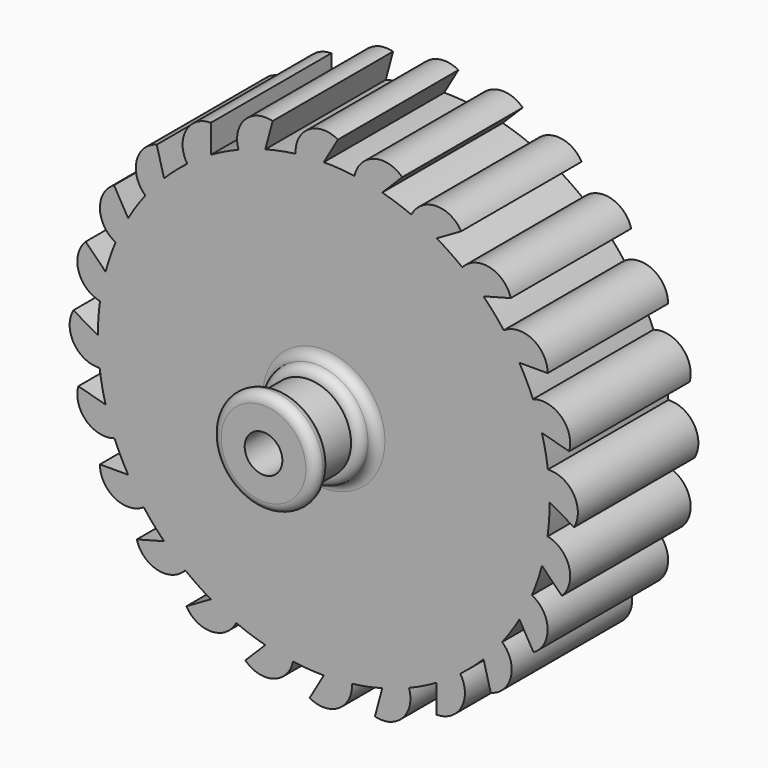
from build123d import *

# Parameters (mm, degrees)
F1_DEPTH  = 50.8
F2_R      = 17.4625
F3_DEPTH  = 6.35
F4_R      = 14.2875
F5_DEPTH  = 12.7
F6_R      = 17.4625
F7_DEPTH  = 6.35
F8_R      = 3.17499
F9_R      = 6.35
F10_DEPTH = 76.201
F11_DEPTH = 25.4


# Not quite as in the source:
# - a fillet or chamfer is up to 0.001 mm smaller than in the source, because OpenCascade refuses the exact size


with BuildPart() as f1:
    # F0 (on Front) → F1 (new body)
    with BuildSketch(Plane.XZ):
        with BuildLine():
            ThreePointArc((-56.346788131, 63.0819802218), (-63.1545591102, 56.0579284352), (-60.182611768, 46.7385626735))
            ThreePointArc((-60.182611768, 46.7385626735), (-63.234562014, 42.5185861347), (-65.9911357684, 38.1))
            Line((-65.9911357684, 38.1), (-70.7536357684, 46.348891971))
            ThreePointArc((-70.7536357684, 46.348891971), (-75.5114792005, 37.8021981611), (-70.2287691608, 29.5695786604))
            ThreePointArc((-70.2287691608, 29.5695786604), (-72.0845164259, 24.7034914868), (-73.6035479632, 19.7220112368))
            Line((-73.6035479632, 19.7220112368), (-80.338740054, 26.4572033276))
            ThreePointArc((-80.338740054, 26.4572033276), (-82.7224167718, 16.9703105533), (-75.4889519939, 10.3854767276))
            ThreePointArc((-75.4889519939, 10.3854767276), (-76.0220301687, 5.2048947186), (-76.2, 0))
            Line((-76.2, 0), (-84.448891971, 4.7625))
            ThreePointArc((-84.448891971, 4.7625), (-84.2959583455, -5.0180756738), (-75.6046875, -9.5063782813))
            ThreePointArc((-75.6046875, -9.5063782813), (-74.7787681878, -14.6484070232), (-73.6035479632, -19.7220112368))
            Line((-73.6035479632, -19.7220112368), (-82.8039914586, -17.2567598322))
            ThreePointArc((-82.8039914586, -17.2567598322), (-80.1248696635, -26.6644883366), (-70.5680884956, -28.7503893204))
            ThreePointArc((-70.5680884956, -28.7503893204), (-68.4394567327, -33.503444034), (-65.9911357684, -38.1))
            Line((-65.9911357684, -38.1), (-75.5161357684, -38.1))
            ThreePointArc((-75.5161357684, -38.1), (-70.4934035266, -46.4937601844), (-60.7223908795, -46.0351088396))
            ThreePointArc((-60.7223908795, -46.0351088396), (-57.4361094027, -50.075276701), (-53.8815367264, -53.8815367264))
            Line((-53.8815367264, -53.8815367264), (-63.0819802218, -56.346788131))
            ThreePointArc((-63.0819802218, -56.346788131), (-56.0579284352, -63.1545591102), (-46.7385626735, -60.182611768))
            ThreePointArc((-46.7385626735, -60.182611768), (-42.5185861347, -63.234562014), (-38.1, -65.9911357684))
            Line((-38.1, -65.9911357684), (-46.348891971, -70.7536357684))
            ThreePointArc((-46.348891971, -70.7536357684), (-37.8021981611, -75.5114792005), (-29.5695786604, -70.2287691608))
            ThreePointArc((-29.5695786604, -70.2287691608), (-24.7034914868, -72.0845164259), (-19.7220112368, -73.6035479632))
            Line((-19.7220112368, -73.6035479632), (-26.4572033276, -80.338740054))
            ThreePointArc((-26.4572033276, -80.338740054), (-16.9703105533, -82.7224167718), (-10.3854767276, -75.4889519939))
            ThreePointArc((-10.3854767276, -75.4889519939), (-5.2048947186, -76.0220301687), (0, -76.2))
            Line((0, -76.2), (-4.7625, -84.448891971))
            ThreePointArc((-4.7625, -84.448891971), (5.0180756738, -84.2959583455), (9.5063782813, -75.6046875))
            ThreePointArc((9.5063782813, -75.6046875), (14.6484070232, -74.7787681878), (19.7220112368, -73.6035479632))
            Line((19.7220112368, -73.6035479632), (17.2567598322, -82.8039914586))
            ThreePointArc((17.2567598322, -82.8039914586), (26.6644883366, -80.1248696635), (28.7503893204, -70.5680884956))
            ThreePointArc((28.7503893204, -70.5680884956), (33.503444034, -68.4394567327), (38.1, -65.9911357684))
            Line((38.1, -65.9911357684), (38.1, -75.5161357684))
            ThreePointArc((38.1, -75.5161357684), (46.4937601844, -70.4934035266), (46.0351088396, -60.7223908795))
            ThreePointArc((46.0351088396, -60.7223908795), (50.075276701, -57.4361094027), (53.8815367264, -53.8815367264))
            Line((53.8815367264, -53.8815367264), (56.346788131, -63.0819802218))
            ThreePointArc((56.346788131, -63.0819802218), (63.1545591102, -56.0579284352), (60.182611768, -46.7385626735))
            ThreePointArc((60.182611768, -46.7385626735), (63.234562014, -42.5185861347), (65.9911357684, -38.1))
            Line((65.9911357684, -38.1), (70.7536357684, -46.348891971))
            ThreePointArc((70.7536357684, -46.348891971), (75.5114792005, -37.8021981611), (70.2287691608, -29.5695786604))
            ThreePointArc((70.2287691608, -29.5695786604), (72.0845164259, -24.7034914868), (73.6035479632, -19.7220112368))
            Line((73.6035479632, -19.7220112368), (80.338740054, -26.4572033276))
            ThreePointArc((80.338740054, -26.4572033276), (82.7224167718, -16.9703105533), (75.4889519939, -10.3854767276))
            ThreePointArc((75.4889519939, -10.3854767276), (76.0220301687, -5.2048947186), (76.2, 0))
            Line((76.2, 0), (84.448891971, -4.7625))
            ThreePointArc((84.448891971, -4.7625), (84.2959583455, 5.0180756738), (75.6046875, 9.5063782813))
            ThreePointArc((75.6046875, 9.5063782813), (74.7787681878, 14.6484070232), (73.6035479632, 19.7220112368))
            Line((73.6035479632, 19.7220112368), (82.8039914586, 17.2567598322))
            ThreePointArc((82.8039914586, 17.2567598322), (80.1248696635, 26.6644883366), (70.5680884956, 28.7503893204))
            ThreePointArc((70.5680884956, 28.7503893204), (68.4394567327, 33.503444034), (65.9911357684, 38.1))
            Line((65.9911357684, 38.1), (75.5161357684, 38.1))
            ThreePointArc((75.5161357684, 38.1), (70.4934035266, 46.4937601844), (60.7223908795, 46.0351088396))
            ThreePointArc((60.7223908795, 46.0351088396), (57.4361094027, 50.075276701), (53.8815367264, 53.8815367264))
            Line((53.8815367264, 53.8815367264), (63.0819802218, 56.346788131))
            ThreePointArc((63.0819802218, 56.346788131), (56.0579284352, 63.1545591102), (46.7385626735, 60.182611768))
            ThreePointArc((46.7385626735, 60.182611768), (42.5185861347, 63.234562014), (38.1, 65.9911357684))
            Line((38.1, 65.9911357684), (46.348891971, 70.7536357684))
            ThreePointArc((46.348891971, 70.7536357684), (37.8021981611, 75.5114792005), (29.5695786604, 70.2287691608))
            ThreePointArc((29.5695786604, 70.2287691608), (24.7034914868, 72.0845164259), (19.7220112368, 73.6035479632))
            Line((19.7220112368, 73.6035479632), (26.4572033276, 80.338740054))
            ThreePointArc((26.4572033276, 80.338740054), (16.9703105533, 82.7224167718), (10.3854767276, 75.4889519939))
            ThreePointArc((10.3854767276, 75.4889519939), (5.2048947186, 76.0220301687), (0, 76.2))
            Line((0, 76.2), (4.7625, 84.448891971))
            ThreePointArc((4.7625, 84.448891971), (-5.0180756738, 84.2959583455), (-9.5063782813, 75.6046875))
            ThreePointArc((-9.5063782813, 75.6046875), (-14.6484070232, 74.7787681878), (-19.7220112368, 73.6035479632))
            Line((-19.7220112368, 73.6035479632), (-17.2567598322, 82.8039914586))
            ThreePointArc((-17.2567598322, 82.8039914586), (-26.6644883366, 80.1248696635), (-28.7503893204, 70.5680884956))
            ThreePointArc((-28.7503893204, 70.5680884956), (-33.503444034, 68.4394567327), (-38.1, 65.9911357684))
            Line((-38.1, 65.9911357684), (-38.1, 75.5161357684))
            ThreePointArc((-38.1, 75.5161357684), (-46.4937601844, 70.4934035266), (-46.0351088396, 60.7223908795))
            ThreePointArc((-46.0351088396, 60.7223908795), (-50.075276701, 57.4361094027), (-53.8815367264, 53.8815367264))
            Line((-53.8815367264, 53.8815367264), (-56.346788131, 63.0819802218))
        make_face()
    extrude(amount=F1_DEPTH)

    # F2 (on face) → F3 (join)
    with BuildSketch(Plane.XZ.offset(50.8)):
        Circle(F2_R)
    extrude(amount=F3_DEPTH)

    # F4 (on face) → F5 (join)
    with BuildSketch(Plane.XZ.offset(57.15)):
        Circle(F4_R)
    extrude(amount=F5_DEPTH)

    # F6 (on face) → F7 (join)
    with BuildSketch(Plane.XZ.offset(69.85)):
        Circle(F6_R)
    extrude(amount=F7_DEPTH)

    # F8 (radius 3.175 in the source; OpenCascade refuses exactly that, so slightly less here)
    f8_edges = [f1.edges().sort_by_distance(p)[0] for p in [
        (17.4625, -53.975, 0),
        (-17.4625, -50.8, 0),
        (-17.4625, -57.15, 0),
        (17.4625, -73.025, 0),
        (-17.4625, -69.85, 0),
        (-17.4625, -76.2, 0),
    ]]
    fillet(f8_edges, radius=F8_R)

    # F9 (on face) → F10 (cut, through all)
    with BuildSketch(Plane.XZ.offset(76.2)):
        Circle(F9_R)
    extrude(amount=-F10_DEPTH, mode=Mode.SUBTRACT)

    # F0 (on Front) → F11 (join)
    with BuildSketch(Plane.XZ):
        with BuildLine():
            ThreePointArc((-56.346788131, 63.0819802218), (-63.1545591102, 56.0579284352), (-60.182611768, 46.7385626735))
            ThreePointArc((-60.182611768, 46.7385626735), (-63.234562014, 42.5185861347), (-65.9911357684, 38.1))
            Line((-65.9911357684, 38.1), (-70.7536357684, 46.348891971))
            ThreePointArc((-70.7536357684, 46.348891971), (-75.5114792005, 37.8021981611), (-70.2287691608, 29.5695786604))
            ThreePointArc((-70.2287691608, 29.5695786604), (-72.0845164259, 24.7034914868), (-73.6035479632, 19.7220112368))
            Line((-73.6035479632, 19.7220112368), (-80.338740054, 26.4572033276))
            ThreePointArc((-80.338740054, 26.4572033276), (-82.7224167718, 16.9703105533), (-75.4889519939, 10.3854767276))
            ThreePointArc((-75.4889519939, 10.3854767276), (-76.0220301687, 5.2048947186), (-76.2, 0))
            Line((-76.2, 0), (-84.448891971, 4.7625))
            ThreePointArc((-84.448891971, 4.7625), (-84.2959583455, -5.0180756738), (-75.6046875, -9.5063782813))
            ThreePointArc((-75.6046875, -9.5063782813), (-74.7787681878, -14.6484070232), (-73.6035479632, -19.7220112368))
            Line((-73.6035479632, -19.7220112368), (-82.8039914586, -17.2567598322))
            ThreePointArc((-82.8039914586, -17.2567598322), (-80.1248696635, -26.6644883366), (-70.5680884956, -28.7503893204))
            ThreePointArc((-70.5680884956, -28.7503893204), (-68.4394567327, -33.503444034), (-65.9911357684, -38.1))
            Line((-65.9911357684, -38.1), (-75.5161357684, -38.1))
            ThreePointArc((-75.5161357684, -38.1), (-70.4934035266, -46.4937601844), (-60.7223908795, -46.0351088396))
            ThreePointArc((-60.7223908795, -46.0351088396), (-57.4361094027, -50.075276701), (-53.8815367264, -53.8815367264))
            Line((-53.8815367264, -53.8815367264), (-63.0819802218, -56.346788131))
            ThreePointArc((-63.0819802218, -56.346788131), (-56.0579284352, -63.1545591102), (-46.7385626735, -60.182611768))
            ThreePointArc((-46.7385626735, -60.182611768), (-42.5185861347, -63.234562014), (-38.1, -65.9911357684))
            Line((-38.1, -65.9911357684), (-46.348891971, -70.7536357684))
            ThreePointArc((-46.348891971, -70.7536357684), (-37.8021981611, -75.5114792005), (-29.5695786604, -70.2287691608))
            ThreePointArc((-29.5695786604, -70.2287691608), (-24.7034914868, -72.0845164259), (-19.7220112368, -73.6035479632))
            Line((-19.7220112368, -73.6035479632), (-26.4572033276, -80.338740054))
            ThreePointArc((-26.4572033276, -80.338740054), (-16.9703105533, -82.7224167718), (-10.3854767276, -75.4889519939))
            ThreePointArc((-10.3854767276, -75.4889519939), (-5.2048947186, -76.0220301687), (0, -76.2))
            Line((0, -76.2), (-4.7625, -84.448891971))
            ThreePointArc((-4.7625, -84.448891971), (5.0180756738, -84.2959583455), (9.5063782813, -75.6046875))
            ThreePointArc((9.5063782813, -75.6046875), (14.6484070232, -74.7787681878), (19.7220112368, -73.6035479632))
            Line((19.7220112368, -73.6035479632), (17.2567598322, -82.8039914586))
            ThreePointArc((17.2567598322, -82.8039914586), (26.6644883366, -80.1248696635), (28.7503893204, -70.5680884956))
            ThreePointArc((28.7503893204, -70.5680884956), (33.503444034, -68.4394567327), (38.1, -65.9911357684))
            Line((38.1, -65.9911357684), (38.1, -75.5161357684))
            ThreePointArc((38.1, -75.5161357684), (46.4937601844, -70.4934035266), (46.0351088396, -60.7223908795))
            ThreePointArc((46.0351088396, -60.7223908795), (50.075276701, -57.4361094027), (53.8815367264, -53.8815367264))
            Line((53.8815367264, -53.8815367264), (56.346788131, -63.0819802218))
            ThreePointArc((56.346788131, -63.0819802218), (63.1545591102, -56.0579284352), (60.182611768, -46.7385626735))
            ThreePointArc((60.182611768, -46.7385626735), (63.234562014, -42.5185861347), (65.9911357684, -38.1))
            Line((65.9911357684, -38.1), (70.7536357684, -46.348891971))
            ThreePointArc((70.7536357684, -46.348891971), (75.5114792005, -37.8021981611), (70.2287691608, -29.5695786604))
            ThreePointArc((70.2287691608, -29.5695786604), (72.0845164259, -24.7034914868), (73.6035479632, -19.7220112368))
            Line((73.6035479632, -19.7220112368), (80.338740054, -26.4572033276))
            ThreePointArc((80.338740054, -26.4572033276), (82.7224167718, -16.9703105533), (75.4889519939, -10.3854767276))
            ThreePointArc((75.4889519939, -10.3854767276), (76.0220301687, -5.2048947186), (76.2, 0))
            Line((76.2, 0), (84.448891971, -4.7625))
            ThreePointArc((84.448891971, -4.7625), (84.2959583455, 5.0180756738), (75.6046875, 9.5063782813))
            ThreePointArc((75.6046875, 9.5063782813), (74.7787681878, 14.6484070232), (73.6035479632, 19.7220112368))
            Line((73.6035479632, 19.7220112368), (82.8039914586, 17.2567598322))
            ThreePointArc((82.8039914586, 17.2567598322), (80.1248696635, 26.6644883366), (70.5680884956, 28.7503893204))
            ThreePointArc((70.5680884956, 28.7503893204), (68.4394567327, 33.503444034), (65.9911357684, 38.1))
            Line((65.9911357684, 38.1), (75.5161357684, 38.1))
            ThreePointArc((75.5161357684, 38.1), (70.4934035266, 46.4937601844), (60.7223908795, 46.0351088396))
            ThreePointArc((60.7223908795, 46.0351088396), (57.4361094027, 50.075276701), (53.8815367264, 53.8815367264))
            Line((53.8815367264, 53.8815367264), (63.0819802218, 56.346788131))
            ThreePointArc((63.0819802218, 56.346788131), (56.0579284352, 63.1545591102), (46.7385626735, 60.182611768))
            ThreePointArc((46.7385626735, 60.182611768), (42.5185861347, 63.234562014), (38.1, 65.9911357684))
            Line((38.1, 65.9911357684), (46.348891971, 70.7536357684))
            ThreePointArc((46.348891971, 70.7536357684), (37.8021981611, 75.5114792005), (29.5695786604, 70.2287691608))
            ThreePointArc((29.5695786604, 70.2287691608), (24.7034914868, 72.0845164259), (19.7220112368, 73.6035479632))
            Line((19.7220112368, 73.6035479632), (26.4572033276, 80.338740054))
            ThreePointArc((26.4572033276, 80.338740054), (16.9703105533, 82.7224167718), (10.3854767276, 75.4889519939))
            ThreePointArc((10.3854767276, 75.4889519939), (5.2048947186, 76.0220301687), (0, 76.2))
            Line((0, 76.2), (4.7625, 84.448891971))
            ThreePointArc((4.7625, 84.448891971), (-5.0180756738, 84.2959583455), (-9.5063782813, 75.6046875))
            ThreePointArc((-9.5063782813, 75.6046875), (-14.6484070232, 74.7787681878), (-19.7220112368, 73.6035479632))
            Line((-19.7220112368, 73.6035479632), (-17.2567598322, 82.8039914586))
            ThreePointArc((-17.2567598322, 82.8039914586), (-26.6644883366, 80.1248696635), (-28.7503893204, 70.5680884956))
            ThreePointArc((-28.7503893204, 70.5680884956), (-33.503444034, 68.4394567327), (-38.1, 65.9911357684))
            Line((-38.1, 65.9911357684), (-38.1, 75.5161357684))
            ThreePointArc((-38.1, 75.5161357684), (-46.4937601844, 70.4934035266), (-46.0351088396, 60.7223908795))
            ThreePointArc((-46.0351088396, 60.7223908795), (-50.075276701, 57.4361094027), (-53.8815367264, 53.8815367264))
            Line((-53.8815367264, 53.8815367264), (-56.346788131, 63.0819802218))
        make_face()
    extrude(amount=F11_DEPTH)


solid = f1.part
